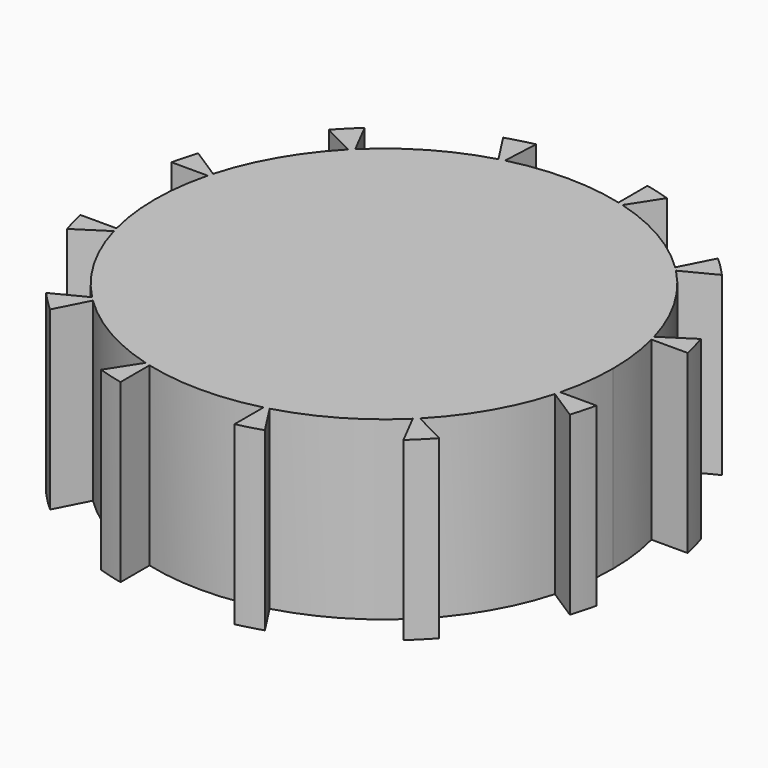
from build123d import *

# Parameters (mm, degrees)
F1_DEPTH = 25.4


# Not quite as in the source:
# - a feature names something its author has since deleted; it is built from what else it names


with BuildPart() as f1:
    # F0 (on Top) → F1 (new body)
    with BuildSketch(Plane.XY):
        with BuildLine():
            Line((31.981135327, 8.217504682), (37.2032608356, 8.217504682))
            ThreePointArc((37.2032608356, 8.217504682), (36.7578953368, 10.0233293076), (36.2249315604, 11.8052671906))
            Line((36.2249315604, 11.8052671906), (31.7868036802, 8.9397713505))
            ThreePointArc((31.7868036802, 8.9397713505), (31.8860146238, 8.5791882723), (31.981135327, 8.217504682))
        make_face()
        with BuildLine():
            ThreePointArc((36.2249315604, -11.8052671906), (36.7578953368, -10.0233293076), (37.2032608356, -8.217504682))
            Line((37.2032608356, -8.217504682), (31.981135327, -8.217504682))
            ThreePointArc((31.981135327, -8.217504682), (31.8860146238, -8.5791882723), (31.7868036802, -8.9397713505))
            Line((31.7868036802, -8.9397713505), (36.2249315604, -11.8052671906))
        make_face()
        with BuildLine():
            ThreePointArc((33.02, 0), (32.7592543299, 4.1414557527), (31.981135327, 8.217504682))
            Line((31.981135327, 8.217504682), (30.6681449847, 8.217504682))
            ThreePointArc((30.6681449847, 8.217504682), (31.4783743486, 4.144206603), (31.75, 0))
            ThreePointArc((31.75, 0), (31.4783743486, -4.144206603), (30.6681449847, -8.217504682))
            Line((30.6681449847, -8.217504682), (31.981135327, -8.217504682))
            ThreePointArc((31.981135327, -8.217504682), (32.7592543299, -4.1414557527), (33.02, 0))
        make_face()
        with BuildLine():
            Line((30.6681449847, 8.217504682), (31.981135327, 8.217504682))
            ThreePointArc((31.981135327, 8.217504682), (31.8860146238, 8.5791882723), (31.7868036802, 8.9397713505))
            Line((31.7868036802, 8.9397713505), (30.6681449847, 8.217504682))
        make_face()
        with BuildLine():
            ThreePointArc((31.7868036802, -8.9397713505), (31.8860146238, -8.5791882723), (31.981135327, -8.217504682))
            Line((31.981135327, -8.217504682), (30.6681449847, -8.217504682))
            Line((30.6681449847, -8.217504682), (31.7868036802, -8.9397713505))
        make_face()
        with BuildLine():
            Line((23.6354709336, 23.0582938169), (28.3361270657, 25.4690773864))
            ThreePointArc((28.3361270657, 25.4690773864), (26.9407683632, 26.9407683632), (25.4690773864, 28.3361270657))
            Line((25.4690773864, 28.3361270657), (23.0582938169, 23.6354709336))
            ThreePointArc((23.0582938169, 23.6354709336), (23.3486659148, 23.3486659148), (23.6354709336, 23.0582938169))
        make_face()
        with BuildLine():
            Line((30.6681449847, 8.217504682), (31.7868036802, 8.9397713505))
            ThreePointArc((31.7868036802, 8.9397713505), (28.596158833, 16.51), (23.6354709336, 23.0582938169))
            Line((23.6354709336, 23.0582938169), (22.4506403027, 22.4506403027))
            ThreePointArc((22.4506403027, 22.4506403027), (27.4963065702, 15.875), (30.6681449847, 8.217504682))
        make_face()
        with BuildLine():
            ThreePointArc((31.75, 0), (31.4783743486, 4.144206603), (30.6681449847, 8.217504682))
            ThreePointArc((30.6681449847, 8.217504682), (27.4963065702, 15.875), (22.4506403027, 22.4506403027))
            ThreePointArc((22.4506403027, 22.4506403027), (15.875, 27.4963065702), (8.217504682, 30.6681449847))
            ThreePointArc((8.217504682, 30.6681449847), (0, 31.75), (-8.217504682, 30.6681449847))
            ThreePointArc((-8.217504682, 30.6681449847), (-15.875, 27.4963065702), (-22.4506403027, 22.4506403027))
            ThreePointArc((-22.4506403027, 22.4506403027), (-27.4963065702, 15.875), (-30.6681449847, 8.217504682))
            ThreePointArc((-30.6681449847, 8.217504682), (-31.75, 0), (-30.6681449847, -8.217504682))
            ThreePointArc((-30.6681449847, -8.217504682), (-27.4963065702, -15.875), (-22.4506403027, -22.4506403027))
            ThreePointArc((-22.4506403027, -22.4506403027), (-15.875, -27.4963065702), (-8.217504682, -30.6681449847))
            ThreePointArc((-8.217504682, -30.6681449847), (0, -31.75), (8.217504682, -30.6681449847))
            ThreePointArc((8.217504682, -30.6681449847), (15.875, -27.4963065702), (22.4506403027, -22.4506403027))
            ThreePointArc((22.4506403027, -22.4506403027), (27.4963065702, -15.875), (30.6681449847, -8.217504682))
            ThreePointArc((30.6681449847, -8.217504682), (31.4783743486, -4.144206603), (31.75, 0))
        make_face()
        with BuildLine():
            ThreePointArc((25.4690773864, -28.3361270657), (26.9407683632, -26.9407683632), (28.3361270657, -25.4690773864))
            Line((28.3361270657, -25.4690773864), (23.6354709336, -23.0582938169))
            ThreePointArc((23.6354709336, -23.0582938169), (23.3486659148, -23.3486659148), (23.0582938169, -23.6354709336))
            Line((23.0582938169, -23.6354709336), (25.4690773864, -28.3361270657))
        make_face()
        with BuildLine():
            ThreePointArc((23.6354709336, -23.0582938169), (28.596158833, -16.51), (31.7868036802, -8.9397713505))
            Line((31.7868036802, -8.9397713505), (30.6681449847, -8.217504682))
            ThreePointArc((30.6681449847, -8.217504682), (27.4963065702, -15.875), (22.4506403027, -22.4506403027))
            Line((22.4506403027, -22.4506403027), (23.6354709336, -23.0582938169))
        make_face()
        with BuildLine():
            Line((22.4506403027, 22.4506403027), (23.6354709336, 23.0582938169))
            ThreePointArc((23.6354709336, 23.0582938169), (23.3486659148, 23.3486659148), (23.0582938169, 23.6354709336))
            Line((23.0582938169, 23.6354709336), (22.4506403027, 22.4506403027))
        make_face()
        with BuildLine():
            ThreePointArc((8.217504682, 30.6681449847), (15.875, 27.4963065702), (22.4506403027, 22.4506403027))
            Line((22.4506403027, 22.4506403027), (23.0582938169, 23.6354709336))
            ThreePointArc((23.0582938169, 23.6354709336), (16.51, 28.596158833), (8.9397713505, 31.7868036802))
            Line((8.9397713505, 31.7868036802), (8.217504682, 30.6681449847))
        make_face()
        with BuildLine():
            ThreePointArc((23.0582938169, -23.6354709336), (23.3486659148, -23.3486659148), (23.6354709336, -23.0582938169))
            Line((23.6354709336, -23.0582938169), (22.4506403027, -22.4506403027))
            Line((22.4506403027, -22.4506403027), (23.0582938169, -23.6354709336))
        make_face()
        with BuildLine():
            Line((23.0582938169, -23.6354709336), (22.4506403027, -22.4506403027))
            ThreePointArc((22.4506403027, -22.4506403027), (15.875, -27.4963065702), (8.217504682, -30.6681449847))
            Line((8.217504682, -30.6681449847), (8.9397713505, -31.7868036802))
            ThreePointArc((8.9397713505, -31.7868036802), (16.51, -28.596158833), (23.0582938169, -23.6354709336))
        make_face()
        with BuildLine():
            Line((8.9397713505, 31.7868036802), (11.8052671906, 36.2249315604))
            ThreePointArc((11.8052671906, 36.2249315604), (10.0233293076, 36.7578953368), (8.217504682, 37.2032608356))
            Line((8.217504682, 37.2032608356), (8.217504682, 31.981135327))
            ThreePointArc((8.217504682, 31.981135327), (8.5791882723, 31.8860146238), (8.9397713505, 31.7868036802))
        make_face()
        with BuildLine():
            Line((8.217504682, 31.981135327), (8.217504682, 30.6681449847))
            Line((8.217504682, 30.6681449847), (8.9397713505, 31.7868036802))
            ThreePointArc((8.9397713505, 31.7868036802), (8.5791882723, 31.8860146238), (8.217504682, 31.981135327))
        make_face()
        with BuildLine():
            ThreePointArc((-8.217504682, 30.6681449847), (0, 31.75), (8.217504682, 30.6681449847))
            Line((8.217504682, 30.6681449847), (8.217504682, 31.981135327))
            ThreePointArc((8.217504682, 31.981135327), (0.0341516637, 33.0199823389), (-8.1513327465, 31.9980651674))
            Line((-8.1513327465, 31.9980651674), (-8.217504682, 30.6681449847))
        make_face()
        with BuildLine():
            ThreePointArc((8.217504682, -37.2032608356), (10.0233293076, -36.7578953368), (11.8052671906, -36.2249315604))
            Line((11.8052671906, -36.2249315604), (8.9397713505, -31.7868036802))
            ThreePointArc((8.9397713505, -31.7868036802), (8.5791882723, -31.8860146238), (8.217504682, -31.981135327))
            Line((8.217504682, -31.981135327), (8.217504682, -37.2032608356))
        make_face()
        with BuildLine():
            Line((8.217504682, -31.981135327), (8.217504682, -30.6681449847))
            ThreePointArc((8.217504682, -30.6681449847), (0, -31.75), (-8.217504682, -30.6681449847))
            Line((-8.217504682, -30.6681449847), (-8.217504682, -31.981135327))
            ThreePointArc((-8.217504682, -31.981135327), (0, -33.02), (8.217504682, -31.981135327))
        make_face()
        with BuildLine():
            Line((8.9397713505, -31.7868036802), (8.217504682, -30.6681449847))
            Line((8.217504682, -30.6681449847), (8.217504682, -31.981135327))
            ThreePointArc((8.217504682, -31.981135327), (8.5791882723, -31.8860146238), (8.9397713505, -31.7868036802))
        make_face()
        with BuildLine():
            Line((-8.9397713505, 31.7868036802), (-8.217504682, 30.6681449847))
            Line((-8.217504682, 30.6681449847), (-8.1513327465, 31.9980651674))
            ThreePointArc((-8.1513327465, 31.9980651674), (-8.5462048693, 31.8948707841), (-8.9397713505, 31.7868036802))
        make_face()
        with BuildLine():
            ThreePointArc((-22.4506403027, 22.4506403027), (-15.875, 27.4963065702), (-8.217504682, 30.6681449847))
            Line((-8.217504682, 30.6681449847), (-8.9397713505, 31.7868036802))
            ThreePointArc((-8.9397713505, 31.7868036802), (-16.51, 28.596158833), (-23.0582938169, 23.6354709336))
            Line((-23.0582938169, 23.6354709336), (-22.4506403027, 22.4506403027))
        make_face()
        with BuildLine():
            Line((-8.9397713505, -31.7868036802), (-8.217504682, -30.6681449847))
            ThreePointArc((-8.217504682, -30.6681449847), (-15.875, -27.4963065702), (-22.4506403027, -22.4506403027))
            Line((-22.4506403027, -22.4506403027), (-23.0582938169, -23.6354709336))
            ThreePointArc((-23.0582938169, -23.6354709336), (-16.51, -28.596158833), (-8.9397713505, -31.7868036802))
        make_face()
        with BuildLine():
            Line((-8.217504682, -31.981135327), (-8.217504682, -30.6681449847))
            Line((-8.217504682, -30.6681449847), (-8.9397713505, -31.7868036802))
            ThreePointArc((-8.9397713505, -31.7868036802), (-8.5791882723, -31.8860146238), (-8.217504682, -31.981135327))
        make_face()
        with BuildLine():
            Line((-8.1513327465, 31.9980651674), (-7.8888044947, 37.274344577))
            ThreePointArc((-7.8888044947, 37.274344577), (-9.8610056184, 36.8017739816), (-11.8052671906, 36.2249315604))
            Line((-11.8052671906, 36.2249315604), (-8.9397713505, 31.7868036802))
            ThreePointArc((-8.9397713505, 31.7868036802), (-8.5462048693, 31.8948707841), (-8.1513327465, 31.9980651674))
        make_face()
        with BuildLine():
            Line((-23.6354709336, 23.0582938169), (-22.4506403027, 22.4506403027))
            Line((-22.4506403027, 22.4506403027), (-23.0582938169, 23.6354709336))
            ThreePointArc((-23.0582938169, 23.6354709336), (-23.3486659148, 23.3486659148), (-23.6354709336, 23.0582938169))
        make_face()
        with BuildLine():
            ThreePointArc((-30.6681449847, 8.217504682), (-27.4963065702, 15.875), (-22.4506403027, 22.4506403027))
            Line((-22.4506403027, 22.4506403027), (-23.6354709336, 23.0582938169))
            ThreePointArc((-23.6354709336, 23.0582938169), (-28.596158833, 16.51), (-31.7868036802, 8.9397713505))
            Line((-31.7868036802, 8.9397713505), (-30.6681449847, 8.217504682))
        make_face()
        with BuildLine():
            ThreePointArc((-11.8052671906, -36.2249315604), (-10.0233293076, -36.7578953368), (-8.217504682, -37.2032608356))
            Line((-8.217504682, -37.2032608356), (-8.217504682, -31.981135327))
            ThreePointArc((-8.217504682, -31.981135327), (-8.5791882723, -31.8860146238), (-8.9397713505, -31.7868036802))
            Line((-8.9397713505, -31.7868036802), (-11.8052671906, -36.2249315604))
        make_face()
        with BuildLine():
            Line((-23.6354709336, -23.0582938169), (-22.4506403027, -22.4506403027))
            ThreePointArc((-22.4506403027, -22.4506403027), (-27.4963065702, -15.875), (-30.6681449847, -8.217504682))
            Line((-30.6681449847, -8.217504682), (-31.7868036802, -8.9397713505))
            ThreePointArc((-31.7868036802, -8.9397713505), (-28.596158833, -16.51), (-23.6354709336, -23.0582938169))
        make_face()
        with BuildLine():
            Line((-23.0582938169, -23.6354709336), (-22.4506403027, -22.4506403027))
            Line((-22.4506403027, -22.4506403027), (-23.6354709336, -23.0582938169))
            ThreePointArc((-23.6354709336, -23.0582938169), (-23.3486659148, -23.3486659148), (-23.0582938169, -23.6354709336))
        make_face()
        with BuildLine():
            Line((-31.981135327, 8.217504682), (-30.6681449847, 8.217504682))
            Line((-30.6681449847, 8.217504682), (-31.7868036802, 8.9397713505))
            ThreePointArc((-31.7868036802, 8.9397713505), (-31.8860146238, 8.5791882723), (-31.981135327, 8.217504682))
        make_face()
        with BuildLine():
            ThreePointArc((-30.6681449847, -8.217504682), (-31.75, 0), (-30.6681449847, 8.217504682))
            Line((-30.6681449847, 8.217504682), (-31.981135327, 8.217504682))
            ThreePointArc((-31.981135327, 8.217504682), (-33.02, 0), (-31.981135327, -8.217504682))
            Line((-31.981135327, -8.217504682), (-30.6681449847, -8.217504682))
        make_face()
        with BuildLine():
            ThreePointArc((-23.6354709336, 23.0582938169), (-23.3486659148, 23.3486659148), (-23.0582938169, 23.6354709336))
            Line((-23.0582938169, 23.6354709336), (-25.4690773864, 28.3361270657))
            ThreePointArc((-25.4690773864, 28.3361270657), (-26.9407683632, 26.9407683632), (-28.3361270657, 25.4690773864))
            Line((-28.3361270657, 25.4690773864), (-23.6354709336, 23.0582938169))
        make_face()
        with BuildLine():
            Line((-31.7868036802, -8.9397713505), (-30.6681449847, -8.217504682))
            Line((-30.6681449847, -8.217504682), (-31.981135327, -8.217504682))
            ThreePointArc((-31.981135327, -8.217504682), (-31.8860146238, -8.5791882723), (-31.7868036802, -8.9397713505))
        make_face()
        with BuildLine():
            Line((-25.4690773864, -28.3361270657), (-23.0582938169, -23.6354709336))
            ThreePointArc((-23.0582938169, -23.6354709336), (-23.3486659148, -23.3486659148), (-23.6354709336, -23.0582938169))
            Line((-23.6354709336, -23.0582938169), (-28.3361270657, -25.4690773864))
            ThreePointArc((-28.3361270657, -25.4690773864), (-26.9407683632, -26.9407683632), (-25.4690773864, -28.3361270657))
        make_face()
        with BuildLine():
            ThreePointArc((-31.981135327, 8.217504682), (-31.8860146238, 8.5791882723), (-31.7868036802, 8.9397713505))
            Line((-31.7868036802, 8.9397713505), (-36.2249315604, 11.8052671906))
            ThreePointArc((-36.2249315604, 11.8052671906), (-36.7578953368, 10.0233293076), (-37.2032608356, 8.217504682))
            Line((-37.2032608356, 8.217504682), (-31.981135327, 8.217504682))
        make_face()
        with BuildLine():
            Line((-36.2249315604, -11.8052671906), (-31.7868036802, -8.9397713505))
            ThreePointArc((-31.7868036802, -8.9397713505), (-31.8860146238, -8.5791882723), (-31.981135327, -8.217504682))
            Line((-31.981135327, -8.217504682), (-37.2032608356, -8.217504682))
            ThreePointArc((-37.2032608356, -8.217504682), (-36.7578953368, -10.0233293076), (-36.2249315604, -11.8052671906))
        make_face()
    extrude(amount=F1_DEPTH)


solid = f1.part
